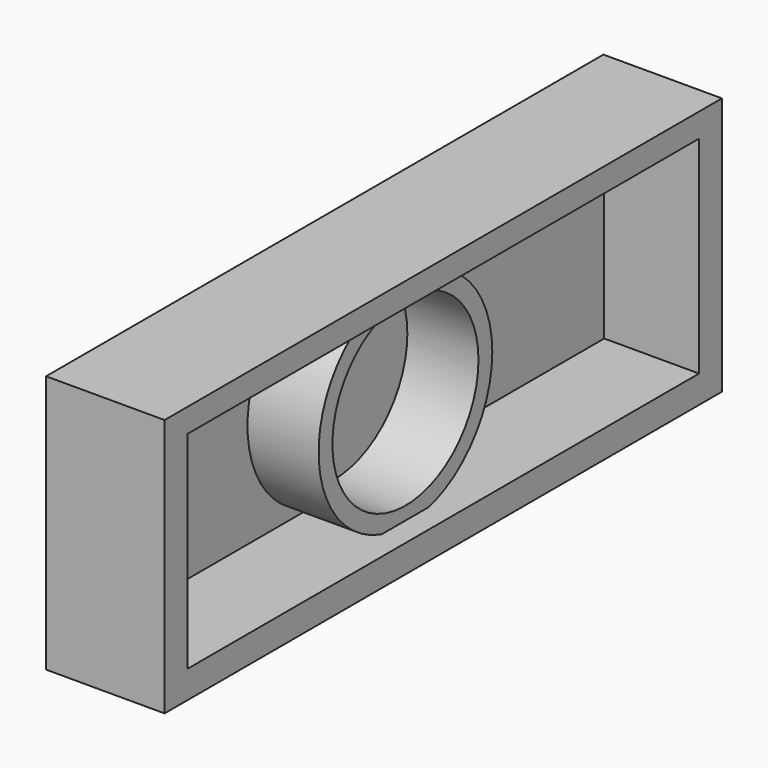
from build123d import *

# Parameters (mm, degrees)
F0_R     = 22.9011210766
F0_R_2   = 19.2527916444
F1_DEPTH = 20
F2_W     = 146.9692662358
F2_H     = 54.4851850718
F2_W_2   = 134.9061205983
F2_H_2   = 43.6283592135
F3_DEPTH = 25
F4_DEPTH = 5
F6_DEPTH = 2
F7_DEPTH = 4


with BuildPart() as f1:
    # F0 (on Right) → F1 (new body)
    with BuildSketch(Plane.YZ):
        Circle(F0_R)
        Circle(F0_R_2, mode=Mode.SUBTRACT)
    extrude(amount=F1_DEPTH)


with BuildPart() as f3:
    # F2 (on Right) → F3 (new body)
    with BuildSketch(Plane.YZ):
        with Locations((3.7194676697, -0.6031570956)):
            Rectangle(F2_W, F2_H)
        with Locations((3.7194676697, -0.2010511234)):
            Rectangle(F2_W_2, F2_H_2, mode=Mode.SUBTRACT)
    extrude(amount=F3_DEPTH)

    # F2 (on Right) → F4 (join)
    with BuildSketch(Plane.YZ):
        with Locations((3.7194676697, -0.2010511234)):
            Rectangle(F2_W_2, F2_H_2)
    extrude(amount=F4_DEPTH)


with BuildPart() as f6:
    # F5 (on Right) → F6 (new body)
    with BuildSketch(Plane.YZ):
        Polygon((5.7423925027, 11.5296468139), (-14.8046044633, 11.5296468139), (-12.6022289523, 9.3272713029), (3.637760787, 9.3272713029), (3.637760787, -6.7213882353), (5.7423925027, -9.0173501521), align=None)
        Polygon((-12.6022289523, 9.3272713029), (-14.8046044633, 11.5296468139), (-14.8046044633, -9.0173501521), (5.7423925027, -9.0173501521), (3.637760787, -6.7213882353), (-12.6022289523, -6.7213882353), align=None)
    extrude(amount=F6_DEPTH)

    # F5 (on Right) → F7 (join)
    with BuildSketch(Plane.YZ):
        Polygon((3.637760787, 9.3272713029), (-12.6022289523, 9.3272713029), (-8.9644681653, 5.7323685173), (0, 5.7323685173), (0, -3.1264854497), (3.637760787, -6.7213882353), align=None)
        Polygon((-8.9644681653, 5.7323685173), (-12.6022289523, 9.3272713029), (-12.6022289523, -6.7213882353), (3.637760787, -6.7213882353), (0, -3.1264854497), (-8.9644681653, -3.1264854497), align=None)
    extrude(amount=F7_DEPTH)


solid = Compound([f1.part, f3.part, f6.part])
